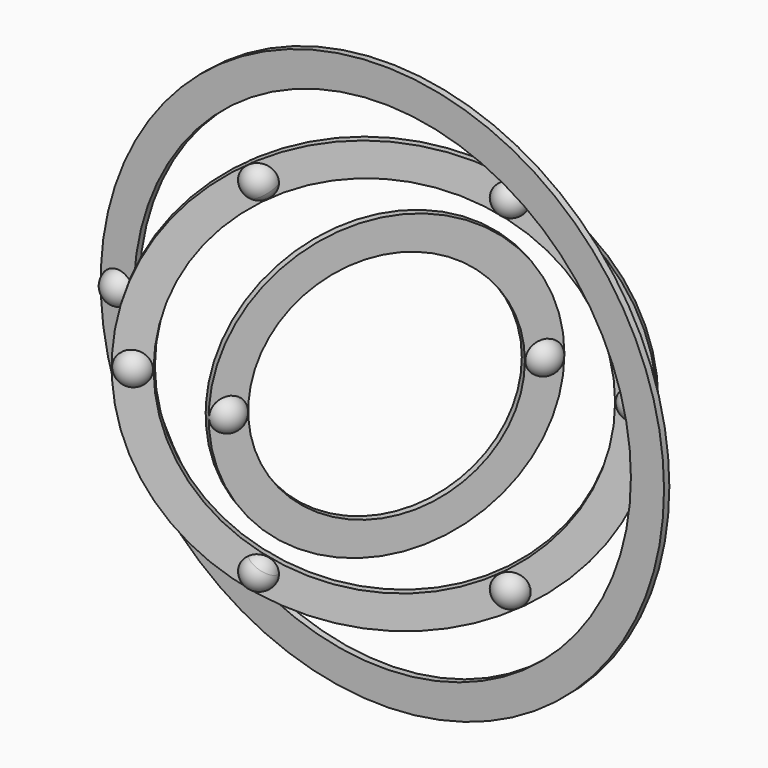
from build123d import *

# Parameters (mm, degrees)
F0_R             = 107.95
F0_R_2           = 95.25
F1_DEPTH         = 1.27
F0_R_3           = 82.55
F0_R_4           = 69.85
F2_DEPTH         = 1.27
F0_R_5           = 57.15
F0_R_6           = 44.45
F3_DEPTH         = 1.27
F4_ANGLE         = 30
F5_ANGLE         = 60
F8_COPIES_COUNT  = 2
F8_COPIES_PITCH  = 41.016833
F8_COPIES1_COUNT = 2
F8_COPIES1_PITCH = 122.848604


# Not quite as in the source:
# - a feature of the source that left no trace in its solid (it failed there, or was rolled back) is left out
# - a pattern or mirror of a feature is missing from the dataset's text; its kind, count and spacing are read off the source's solid


with BuildPart() as f1:
    # F0 (on Front) → F1 (new body, symmetric)
    with BuildSketch(Plane.XZ):
        Circle(F0_R)
        Circle(F0_R_2, mode=Mode.SUBTRACT)
    extrude(amount=F1_DEPTH, both=True)


with BuildPart() as f2:
    # F0 (on Front) → F2 (new body, symmetric)
    with BuildSketch(Plane.XZ):
        Circle(F0_R_3)
        Circle(F0_R_4, mode=Mode.SUBTRACT)
    extrude(amount=F2_DEPTH, both=True)


with BuildPart() as f3:
    # F0 (on Front) → F3 (new body, symmetric)
    with BuildSketch(Plane.XZ):
        Circle(F0_R_5)
        Circle(F0_R_6, mode=Mode.SUBTRACT)
    extrude(amount=F3_DEPTH, both=True)


with BuildPart() as f2_1:
    # F4: moved
    add(f2.part.rotate(Axis((0, 0, 13.3079122752), (0, 0, 1)), F4_ANGLE))


with BuildPart() as f3_1:
    # F5: moved
    add(f3.part.rotate(Axis((0, 0, 13.3079122752), (0, 0, 1)), F5_ANGLE))


with BuildPart() as f8:
    # F7 (on offset) → F8 (revolve)
    with BuildSketch(Plane(origin=(0, 0, 0), x_dir=(0.5, 0.8660254038, 0), z_dir=(0.8660254038, -0.5, 0))):
        with BuildLine():
            ThreePointArc((57.15, 0), (50.8, 6.35), (44.45, 0))
            Line((44.45, 0), (57.15, 0))
        make_face()
    revolve(axis=Axis((-14.2875, -24.7466759131, 0), (-0.5, -0.8660254038, 0)))


with BuildPart() as f8b:
    # F7 (on offset) → F8, piece 2 (revolve)
    with BuildSketch(Plane(origin=(0, 0, 0), x_dir=(0.5, 0.8660254038, 0), z_dir=(0.8660254038, -0.5, 0))):
        with BuildLine():
            Line((-57.15, 0), (-44.45, 0))
            ThreePointArc((-44.45, 0), (-50.8, 6.35), (-57.15, 0))
        make_face()
    revolve(axis=Axis((-14.2875, -24.7466759131, 0), (-0.5, -0.8660254038, 0)))


with BuildPart() as f8_copies_1:
    # F8_copies: instance of F8
    add(f8.part.moved(Location(Vector(0.9896213969, -0.1436993071, 0) * (1 * F8_COPIES_PITCH))))


with BuildPart() as f8_copies1_1:
    # F8_copies1: instance of F8
    add(f8.part.moved(Location(Vector(-0.7439330455, -0.6682541611, 0) * (1 * F8_COPIES1_PITCH))))


with BuildPart() as f12:
    # F10 (on offset) → F12 (revolve)
    with BuildSketch(Plane(origin=(0, 0, 0), x_dir=(0.8660254038, 0.5, 0), z_dir=(0.5, -0.8660254038, 0))):
        with BuildLine():
            ThreePointArc((41.275, -71.4903970824), (43.599261314, -69.1661357684), (44.45, -65.9911357684))
            ThreePointArc((44.45, -65.9911357684), (41.275, -60.4918744543), (34.925, -60.4918744543))
            Line((34.925, -60.4918744543), (41.275, -71.4903970824))
        make_face()
    revolve(axis=Axis((-32.9955678842, -19.05, 65.9911357684), (0.4330127019, 0.25, -0.8660254038)))


with BuildPart() as f12b:
    # F10 (on offset) → F12, piece 2 (revolve)
    with BuildSketch(Plane(origin=(0, 0, 0), x_dir=(0.8660254038, 0.5, 0), z_dir=(0.5, -0.8660254038, 0))):
        with BuildLine():
            ThreePointArc((-34.925, 60.4918744543), (-32.600738686, 62.8161357684), (-31.75, 65.9911357684))
            ThreePointArc((-31.75, 65.9911357684), (-34.925, 71.4903970824), (-41.275, 71.4903970824))
            Line((-41.275, 71.4903970824), (-34.925, 60.4918744543))
        make_face()
    revolve(axis=Axis((-32.9955678842, -19.05, 65.9911357684), (0.4330127019, 0.25, -0.8660254038)))


with BuildPart() as f13:
    # F10 (on offset) → F13 (revolve)
    with BuildSketch(Plane(origin=(0, 0, 0), x_dir=(0.8660254038, 0.5, 0), z_dir=(0.5, -0.8660254038, 0))):
        with BuildLine():
            ThreePointArc((34.925, 60.4918744543), (41.275, 60.4918744543), (44.45, 65.9911357684))
            ThreePointArc((44.45, 65.9911357684), (43.599261314, 69.1661357684), (41.275, 71.4903970824))
            Line((41.275, 71.4903970824), (34.925, 60.4918744543))
        make_face()
    revolve(axis=Axis((32.9955678842, 19.05, 65.9911357684), (-0.4330127019, -0.25, -0.8660254038)))


with BuildPart() as f13b:
    # F10 (on offset) → F13, piece 2 (revolve)
    with BuildSketch(Plane(origin=(0, 0, 0), x_dir=(0.8660254038, 0.5, 0), z_dir=(0.5, -0.8660254038, 0))):
        with BuildLine():
            ThreePointArc((-41.275, -71.4903970824), (-34.925, -71.4903970824), (-31.75, -65.9911357684))
            ThreePointArc((-31.75, -65.9911357684), (-32.600738686, -62.8161357684), (-34.925, -60.4918744543))
            Line((-34.925, -60.4918744543), (-41.275, -71.4903970824))
        make_face()
    revolve(axis=Axis((32.9955678842, 19.05, 65.9911357684), (-0.4330127019, -0.25, -0.8660254038)))


with BuildPart() as f15:
    # F14 (on Front) → F15 (revolve)
    with BuildSketch(Plane.XZ):
        with BuildLine():
            Line((-107.95, 0), (-95.25, 0))
            ThreePointArc((-95.25, 0), (-101.6, 6.35), (-107.95, 0))
        make_face()
    revolve(axis=Axis((-101.6, 0, 0), (1, 0, 0)))


solid = Compound([f1.part, f2_1.part, f3_1.part, f8.part, f8b.part, f8_copies_1.part, f8_copies1_1.part, f12.part, f12b.part, f13.part, f13b.part, f15.part])
